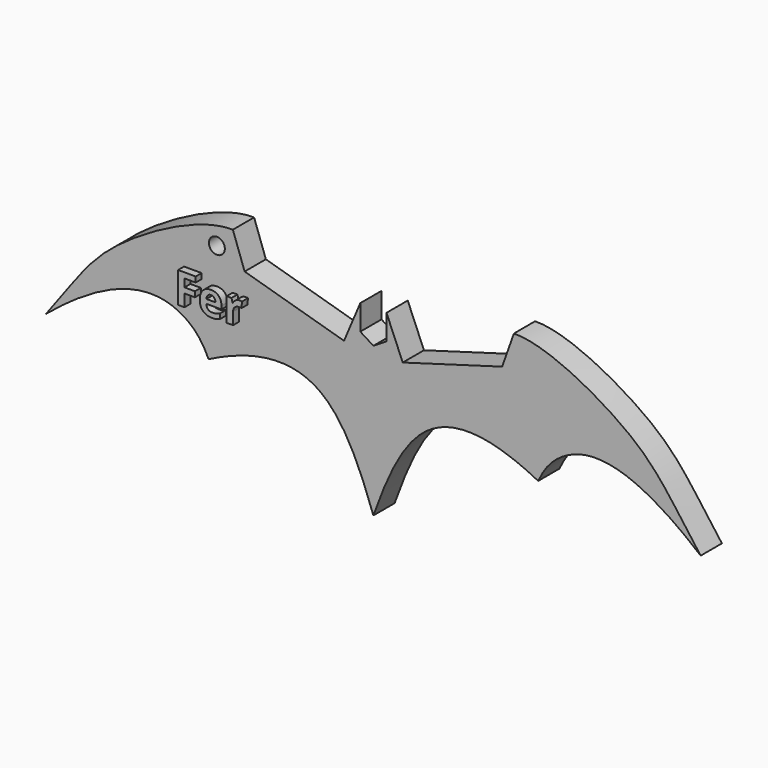
from build123d import *

# Parameters (mm, degrees)
F0_R         = 1.905
F1_DEPTH     = 6.35
F2_TEXT_SIZE = 10.3084047118
F3_DEPTH     = 1.778


# Not quite as in the source:
# - Text() gives the source's letters only with a copy of the font that has no kerning and outlines rounded to 1/6400 em; it was checked with that copy


with BuildPart() as f1:
    # F0 (on Front) → F1 (new body)
    with BuildSketch(Plane.XZ):
        with BuildLine():
            Line((0.811141243, 12.7994463815), (0.811141243, -22.9381090926))
            add(Edge.make_bspline(
                [(0.811141243, -22.9381090926), (4.2133683997, -13.4198734177), (11.7802092108, 4.1628109096), (28.9780276621, 2.9233590735), (40.2374605441, -2.8488031553)],
                knots=[0, 0, 0, 0, 0.4995903231, 1, 1, 1, 1], degree=3))
            add(Edge.make_bspline(
                [(40.2374605441, -2.8488031553), (41.5729606661, 0.1228050323), (46.7196698156, 6.9897359686), (61.2482081052, 8.9777022122), (79.1169846762, -5.9430236887)],
                knots=[0, 0, 0, 0, 0.3412147066, 1, 1, 1, 1], degree=3))
            add(Edge.make_bspline(
                [(34.4281641001, 26.3225012468), (42.2525325287, 26.4419289606), (65.818521701, 13.5881751779), (70.7884263914, 5.2350225006), (79.1169846762, -5.9430236887)],
                knots=[0, 0, 0, 0, 0.5113918248, 1, 1, 1, 1], degree=3))
            Line((34.4281641001, 26.3225012468), (31.6147825474, 18.4204698576))
            Line((31.6147825474, 18.4204698576), (7.8332869129, 11.559051372))
            Line((7.8332869129, 11.559051372), (3.9479141382, 20.7688241854))
            Line((3.9479141382, 20.7688241854), (3.9479141382, 14.7532680108))
            Line((3.9479141382, 14.7532680108), (0.811141243, 12.7994463815))
        make_face()
        with BuildLine():
            add(Edge.make_bspline(
                [(0.811141243, -22.9381090926), (-2.5910859137, -13.4198734177), (-10.1579267248, 4.1628109096), (-27.3557451761, 2.9233590735), (-38.6151780581, -2.8488031553)],
                knots=[0, 0, 0, 0, 0.4995903231, 1, 1, 1, 1], degree=3))
            Line((0.811141243, -22.9381090926), (0.811141243, 12.7994463815))
            Line((0.811141243, 12.7994463815), (-2.3256316522, 14.7532680108))
            Line((-2.3256316522, 14.7532680108), (-2.3256316522, 20.7688241854))
            Line((-2.3256316522, 20.7688241854), (-6.2110044269, 11.559051372))
            Line((-6.2110044269, 11.559051372), (-29.9925000614, 18.4204698576))
            Line((-29.9925000614, 18.4204698576), (-32.8058816141, 26.3225012468))
            add(Edge.make_bspline(
                [(-32.8058816141, 26.3225012468), (-40.6302500427, 26.4419289606), (-64.196239215, 13.5881751779), (-69.1661439054, 5.2350225006), (-77.4947021902, -5.9430236887)],
                knots=[0, 0, 0, 0, 0.5113918248, 1, 1, 1, 1], degree=3))
            add(Edge.make_bspline(
                [(-38.6151780581, -2.8488031553), (-39.9506781801, 0.1228050323), (-45.0973873296, 6.9897359686), (-59.6259256192, 8.9777022122), (-77.4947021902, -5.9430236887)],
                knots=[0, 0, 0, 0, 0.3412147066, 1, 1, 1, 1], degree=3))
        make_face()
        with Locations((-36.6333310699, 21.6878474726)):
            Circle(F0_R, mode=Mode.SUBTRACT)
    extrude(amount=F1_DEPTH)

    # F2 (on face) → F3 (join)
    with BuildSketch(Plane.XZ.offset(6.35)):
        with Locations((-45.4201586545, 7.3978807777)):
            Text('Fer', F2_TEXT_SIZE, font='Open Sans', font_style=FontStyle.BOLD, text_align=(TextAlign.LEFT, TextAlign.BOTTOM))
    extrude(amount=F3_DEPTH)


solid = f1.part
